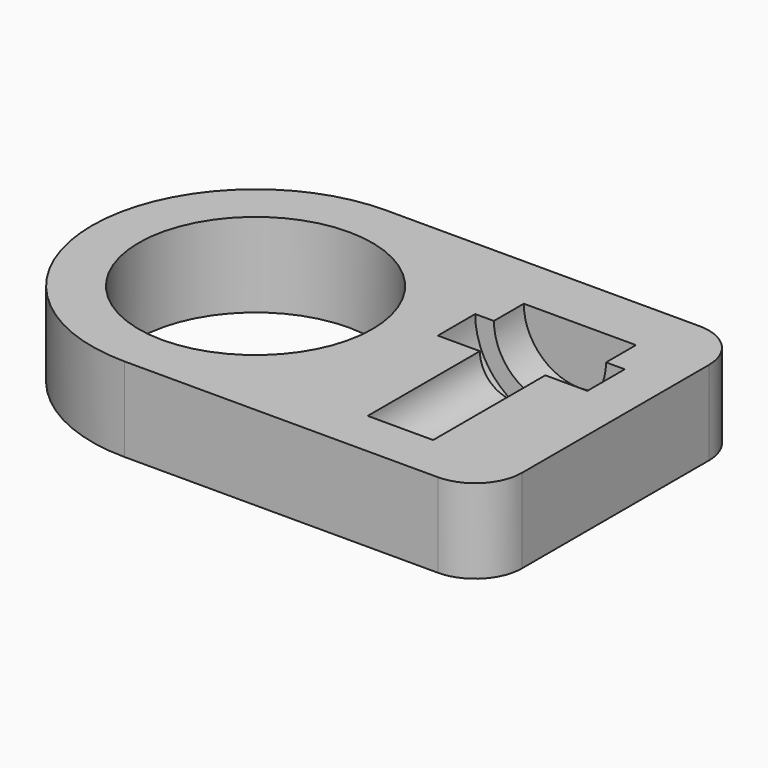
from build123d import *

# Parameters (mm, degrees)
F0_R         = 12.5
F1_DEPTH     = 9
F4_TEXT_SIZE = 5.5555555556
F5_DEPTH     = 1


# Not quite as in the source:
# - Text() gives the source's letters only with a copy of the font that has no kerning and outlines rounded to 1/6400 em; it was checked with that copy


with BuildPart() as f1:
    # F0 (on Top) → F1 (new body)
    with BuildSketch(Plane.XY):
        with BuildLine():
            ThreePointArc((0, 17.5), (5.1256313292, 5.1256313292), (17.5, 0))
            Line((17.5, 0), (51, 0))
            ThreePointArc((51, 0), (54.5355339059, 1.4644660941), (56, 5))
            Line((56, 5), (56, 30))
            ThreePointArc((56, 30), (54.5355339059, 33.5355339059), (51, 35))
            Line((51, 35), (17.5, 35))
            ThreePointArc((17.5, 35), (5.1256313292, 29.8743686708), (0, 17.5))
        make_face()
        with Locations((17.5, 17.5)):
            Circle(F0_R, mode=Mode.SUBTRACT)
    extrude(amount=F1_DEPTH)

    # F2 (on face) → F3 (revolve, cut)
    with BuildSketch(Plane.XY.offset(9)):
        Polygon((43, 20), (43, 5), (46.5, 5), (46.5, 20), (51, 20), (51, 25), (49, 25), (49, 29), (43, 29), (43, 25), align=None)
    revolve(axis=Axis((43, 12.5, 9), (0, 1, 0)), mode=Mode.SUBTRACT)

    # F4 (on face) → F5 (cut)
    with BuildSketch(Plane(origin=(0, 0, 0), x_dir=(1, 0, 0), z_dir=(0, 0, -1))):
        with Locations((30, -9)):
            Text('812', F4_TEXT_SIZE, font='Open Sans', text_align=(TextAlign.LEFT, TextAlign.BOTTOM))
    extrude(amount=-F5_DEPTH, mode=Mode.SUBTRACT)


solid = f1.part
